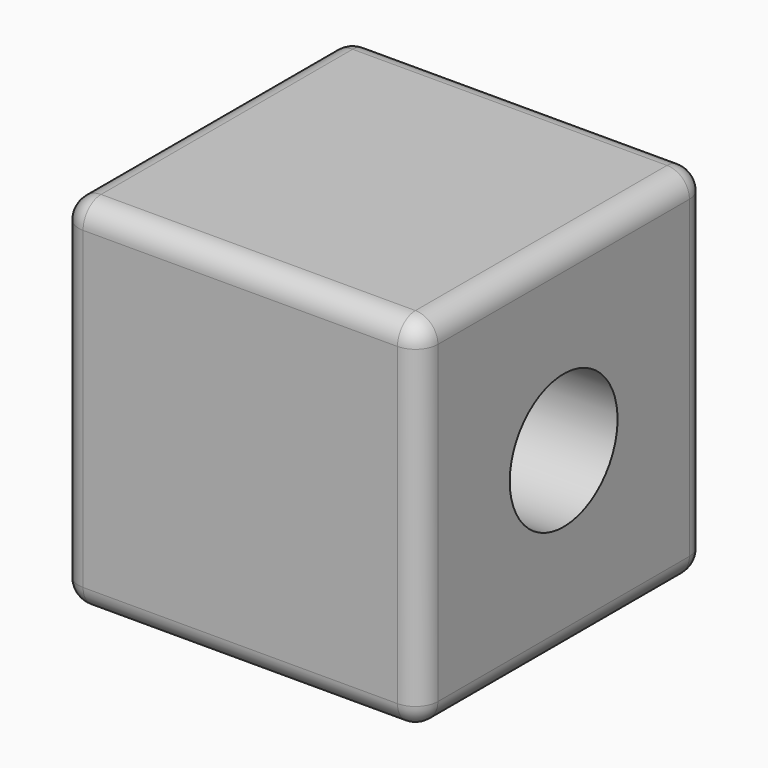
from build123d import *

# Parameters (mm, degrees)
F0_W     = 80
F0_H     = 80
F1_DEPTH = 40
F2_R     = 5
F5_R     = 15
F6_DEPTH = 80.001


# Not quite as in the source:
# - a feature of the source that left no trace in its solid (it failed there, or was rolled back) is left out


with BuildPart() as f1:
    # F0 (on Top) → F1 (new body, symmetric)
    with BuildSketch(Plane.XY):
        Rectangle(F0_W, F0_H)
    extrude(amount=F1_DEPTH, both=True)

    # F2
    f2_edges = [f1.edges().sort_by_distance(p)[0] for p in [
        (40, 0, 40),
        (40, -40, 0),
        (40, 0, -40),
        (40, 40, 0),
        (0, -40, 40),
        (-40, -40, 0),
        (0, -40, -40),
        (-40, 0, 40),
        (0, 40, 40),
        (-40, 0, -40),
        (0, 40, -40),
        (-40, 40, 0),
    ]]
    fillet(f2_edges, radius=F2_R)

    # F5 (on face) → F6 (cut, through all)
    with BuildSketch(Plane(origin=(-40, 0, 0), x_dir=(0, -1, 0), z_dir=(-1, 0, 0))):
        Circle(F5_R)
    extrude(amount=-F6_DEPTH, mode=Mode.SUBTRACT)


solid = f1.part
